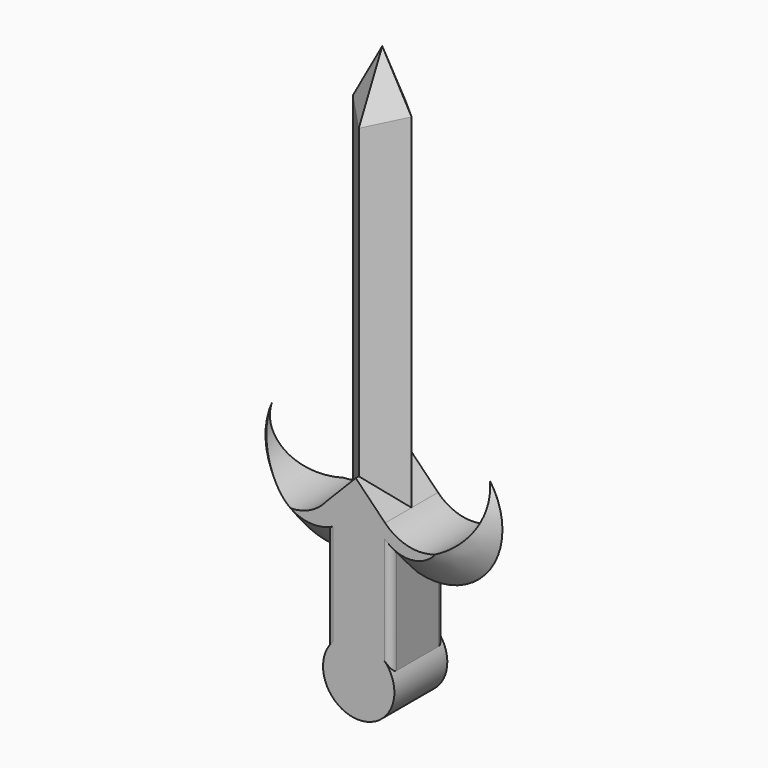
from build123d import *

# Parameters (mm, degrees)
F1_DEPTH    = 10
F2_SIZE     = 4.99999
F3_T1_DEPTH = 67.4287295288
F4_DEPTH    = 10
F5_T4_ANGLE = 302.1740734605
F5_T9_ANGLE = 359.64
F6_T4_ANGLE = 359.64
F6_T9_ANGLE = 302.1740734605
F7_R        = 1


# Not quite as in the source:
# - a fillet or chamfer that OpenCascade refuses, or shapes differently, is made with other operations: its cross-section is extruded or revolved along the edge and cut away or added
# - a fillet or chamfer is up to 0.001 mm smaller than in the source, because OpenCascade refuses the exact size


with BuildPart() as f1:
    # F0 (on Front) → F1 (new body)
    with BuildSketch(Plane.XZ):
        Polygon((35.3119149804, 10.4430096801), (39.7443734109, 5.9087900445), (39.7443734109, 57.9162985086), (35.3119149804, 65.8947229385), (30.8794565499, 57.9162985086), (30.8794565499, 5.9087900445), align=None)
    extrude(amount=F1_DEPTH)

    # F2 (size 5 in the source; OpenCascade refuses exactly that, so slightly less here)
    f2_edges = [f1.edges().sort_by_distance(p)[0] for p in [
        (37.528144, -10, 61.905511),
        (37.528144, 0, 61.905511),
        (33.095686, -10, 61.905511),
        (33.095686, 0, 61.905511),
    ]]
    chamfer(f2_edges, length=F2_SIZE)

    # F3: chamfer of 5 on 4 edges, made by hand

    # F3_s2 → F3_t1 (cut)
    with BuildSketch(Plane.XY.offset(-6.9496248953)):
        Polygon((30.8794565499, -5), (35.8794565499, 0), (30.8794565499, 0), align=None)
        Polygon((30.8794565499, -5), (35.8794565499, -10), (30.8794565499, -10), align=None)
        Polygon((34.7443734109, -10), (39.7443734109, -5), (39.7443734109, -10), align=None)
        Polygon((34.7443734109, 0), (39.7443734109, -5), (39.7443734109, 0), align=None)
    extrude(amount=F3_T1_DEPTH, mode=Mode.SUBTRACT)

    # F0 (on Front) → F4 (join)
    with BuildSketch(Plane.XZ):
        with BuildLine():
            ThreePointArc((51.5925973184, 13.3139307646), (48.6483872163, 4.8435179428), (39.7443734109, 5.9087900445))
            Line((39.7443734109, 5.9087900445), (35.3119149804, 10.4430096801))
            Line((35.3119149804, 10.4430096801), (30.8794565499, 5.9087900445))
            ThreePointArc((30.8794565499, 5.9087900445), (21.5650677315, 4.2615226747), (18.7640711665, 13.2962195203))
            ThreePointArc((18.7640711665, 13.2962195203), (19.9563786111, 1.6237063121), (30.8794565499, -2.6606291067))
            Line((30.8794565499, -2.6606291067), (30.8794565499, -13.8895222917))
            ThreePointArc((30.8794565499, -13.8895222917), (35.755161196, -21.5906926023), (40.6308658421, -13.8895222917))
            Line((40.6308658421, -13.8895222917), (40.6308658421, -2.3651318625))
            ThreePointArc((40.6308658421, -2.3651318625), (51.65255991, 1.6006300969), (51.5925973184, 13.3139307646))
        make_face()
    extrude(amount=F4_DEPTH)

    # F5: chamfer of 5 on 2 edges, made by hand


with BuildPart() as f5_tool2:
    # F5_s3 → F5_t4 (revolve)
    with BuildSketch(Plane(origin=(9.3560149059, 0, -9.9565277283), x_dir=(0, 1, 0), z_dir=(0.6847887183, 0, -0.728741663))):
        Polygon((-10, 33.1289388428), (-5, 38.1289388428), (-10, 38.1289388428), align=None)
    revolve(axis=Axis((28.9307170955, -10, 8.4375560791), (0, -1, 0)), revolution_arc=F5_T4_ANGLE)

    split(bisect_by=Plane.YZ.offset(30.8794565499), keep=Keep.BOTTOM)


with BuildPart() as f1_1:
    add(f1.part)

    # F5_t1: cut F5_tool2
    add(f5_tool2.part, mode=Mode.SUBTRACT)


with BuildPart() as f5_tool7:
    # F5_s8 → F5_t9 (revolve)
    with BuildSketch(Plane(origin=(12.756533571, 0, -16.3882307622), x_dir=(0, 1, 0), z_dir=(-0.6142445443, 0, 0.7891157328))):
        Polygon((-5, -28.604545656), (-10, -33.604545656), (-10, -28.604545656), align=None)
    revolve(axis=Axis((43.3362013883, -10, 7.4148609054), (0, -1, 0)), revolution_arc=F5_T9_ANGLE)

    split(bisect_by=Plane.YZ.offset(40.6308658421), keep=Keep.TOP)


with BuildPart() as f1_2:
    add(f1_1.part)

    # F5_t6: cut F5_tool7
    add(f5_tool7.part, mode=Mode.SUBTRACT)

    # F6: chamfer of 5 on 2 edges, made by hand


with BuildPart() as f6_tool2:
    # F6_s3 → F6_t4 (revolve)
    with BuildSketch(Plane(origin=(12.756533571, 0, -16.3882307622), x_dir=(0, 1, 0), z_dir=(-0.6142445443, 0, 0.7891157328))):
        Polygon((-5, -28.604545656), (0, -33.604545656), (0, -28.604545656), align=None)
    revolve(axis=Axis((43.3362013883, 0, 7.4148609054), (0, -1, 0)), revolution_arc=F6_T4_ANGLE)

    split(bisect_by=Plane.YZ.offset(40.6308658421), keep=Keep.TOP)


with BuildPart() as f1_3:
    add(f1_2.part)

    # F6_t1: cut F6_tool2
    add(f6_tool2.part, mode=Mode.SUBTRACT)


with BuildPart() as f6_tool7:
    # F6_s8 → F6_t9 (revolve)
    with BuildSketch(Plane(origin=(9.3560149059, 0, -9.9565277283), x_dir=(0, 1, 0), z_dir=(0.6847887183, 0, -0.728741663))):
        Polygon((-5, 38.1289388428), (0, 33.1289388428), (0, 38.1289388428), align=None)
    revolve(axis=Axis((28.9307170955, 0, 8.4375560791), (0, -1, 0)), revolution_arc=F6_T9_ANGLE)

    split(bisect_by=Plane.YZ.offset(30.8794565499), keep=Keep.BOTTOM)


with BuildPart() as f1_4:
    add(f1_3.part)

    # F6_t6: cut F6_tool7
    add(f6_tool7.part, mode=Mode.SUBTRACT)

    # F7
    f7_edges = [f1_4.edges().sort_by_distance(p)[0] for p in [
        (40.630866, 0, -5.426826),
        (30.879457, 0, -5.704655),
        (40.630866, -10, -5.426826),
        (30.879457, -10, -5.704655),
    ]]
    fillet(f7_edges, radius=F7_R)


solid = f1_4.part
